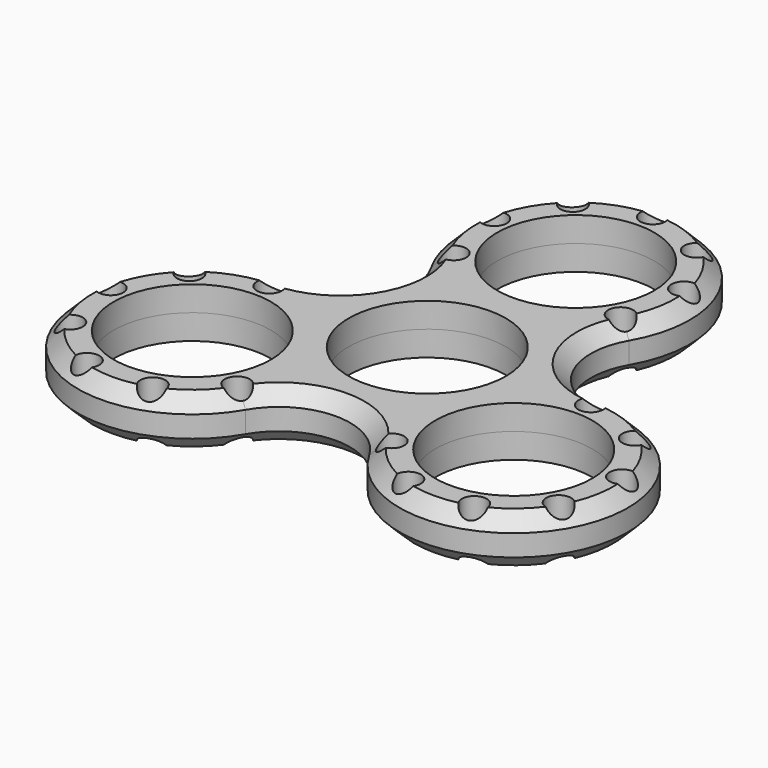
from build123d import *

# Parameters (mm, degrees)
F0_R         = 1.75
F0_R_2       = 11
F1_DEPTH     = 3.5
F2_T2_ANGLE  = 240
F2_T4_ANGLE  = 120
F2_T6_ANGLE  = 240
F2_T8_ANGLE  = 120
F2_T10_ANGLE = 240
F2_T12_ANGLE = 120
F2_T14_ANGLE = 120
F2_T16_ANGLE = 240
F2_T18_ANGLE = 120
F2_T20_ANGLE = 240
F2_T22_ANGLE = 120
F2_T24_ANGLE = 240


# Not quite as in the source:
# - a fillet or chamfer that OpenCascade refuses, or shapes differently, is made with other operations: its cross-section is extruded or revolved along the edge and cut away or added


with BuildPart() as f1:
    # F0 (on Top) → F1 (new body, symmetric)
    with BuildSketch(Plane.XY):
        with BuildLine():
            ThreePointArc((22.5166604984, 3), (13.8564064606, 8), (13.8564064606, 18))
            ThreePointArc((13.8564064606, 18), (0, 42), (-13.8564064606, 18))
            ThreePointArc((-13.8564064606, 18), (-13.8564064606, 8), (-22.5166604984, 3))
            ThreePointArc((-22.5166604984, 3), (-36.3730669589, -21), (-8.6602540378, -21))
            ThreePointArc((-8.6602540378, -21), (0, -16), (8.6602540378, -21))
            ThreePointArc((8.6602540378, -21), (36.3730669589, -21), (22.5166604984, 3))
        make_face()
        with Locations((-27.1339324333, -25.6858503806)):
            Circle(F0_R, mode=Mode.SUBTRACT)
        with Locations((-34.2080034495, -19.75)):
            Circle(F0_R, mode=Mode.SUBTRACT)
        with Locations((-22.5166604984, -13)):
            Circle(F0_R_2, mode=Mode.SUBTRACT)
        with Locations((-17.8993885635, -25.6858503806)):
            Circle(F0_R, mode=Mode.SUBTRACT)
        with Locations((-10.8253175473, -19.75)):
            Circle(F0_R, mode=Mode.SUBTRACT)
        with Locations((-35.8115651641, -10.6557496015)):
            Circle(F0_R, mode=Mode.SUBTRACT)
        with Locations((-31.1942932292, -2.6584000179)):
            Circle(F0_R, mode=Mode.SUBTRACT)
        with Locations((-22.5166604984, 0.5)):
            Circle(F0_R, mode=Mode.SUBTRACT)
        with Locations((17.8993885635, -25.6858503806)):
            Circle(F0_R, mode=Mode.SUBTRACT)
        with Locations((10.8253175473, -19.75)):
            Circle(F0_R, mode=Mode.SUBTRACT)
        with Locations((27.1339324333, -25.6858503806)):
            Circle(F0_R, mode=Mode.SUBTRACT)
        with Locations((22.5166604984, -13)):
            Circle(F0_R_2, mode=Mode.SUBTRACT)
        with Locations((34.2080034495, -19.75)):
            Circle(F0_R, mode=Mode.SUBTRACT)
        Circle(F0_R_2, mode=Mode.SUBTRACT)
        with Locations((35.8115651641, -10.6557496015)):
            Circle(F0_R, mode=Mode.SUBTRACT)
        with Locations((31.1942932292, -2.6584000179)):
            Circle(F0_R, mode=Mode.SUBTRACT)
        with Locations((22.5166604984, 0.5)):
            Circle(F0_R, mode=Mode.SUBTRACT)
        with BuildLine():
            ThreePointArc((-10.1480272234, 18.4249687492), (-13.4411094984, 19.221416266), (-10.1757984945, 20.125))
            ThreePointArc((-10.1757984945, 20.125), (-10.0009727551, 19.7029333289), (-9.9413429511, 19.25))
            ThreePointArc((-9.9413429511, 19.25), (-9.9938002383, 18.8247368599), (-10.1480272234, 18.4249687492))
        make_face(mode=Mode.SUBTRACT)
        with Locations((-13.2949046657, 28.3442503985)):
            Circle(F0_R, mode=Mode.SUBTRACT)
        with Locations((-8.6776327308, 36.3415999821)):
            Circle(F0_R, mode=Mode.SUBTRACT)
        with BuildLine():
            ThreePointArc((10.1480272234, 18.4249687492), (11.266079811, 20.9475427128), (13.4413429511, 19.25))
            ThreePointArc((13.4413429511, 19.25), (12.1166060911, 17.5524572872), (10.1480272234, 18.4249687492))
        make_face(mode=Mode.SUBTRACT)
        with BuildLine():
            ThreePointArc((-9.5262794416, 20.5), (-2.8470094961, 36.6251840892), (11, 26))
            ThreePointArc((11, 26), (2.8470094961, 15.3748159108), (-9.5262794416, 20.5))
        make_face(mode=Mode.SUBTRACT)
        with Locations((13.2949046657, 28.3442503985)):
            Circle(F0_R, mode=Mode.SUBTRACT)
        with Locations((8.6776327308, 36.3415999821)):
            Circle(F0_R, mode=Mode.SUBTRACT)
        with Locations((0, 39.5)):
            Circle(F0_R, mode=Mode.SUBTRACT)
    extrude(amount=F1_DEPTH, both=True)

    # F2: chamfer of 2 on 12 edges, made by hand

    # F2_s1 → F2_t2 (revolve, cut)
    with BuildSketch(Plane.YZ.offset(-22.5166604984)):
        Polygon((3, 1.5), (1, 3.5), (3, 3.5), align=None)
    revolve(axis=Axis((-22.5166604984, -13, 3.5), (0, 0, 1)), revolution_arc=F2_T2_ANGLE, mode=Mode.SUBTRACT)

    # F2_s3 → F2_t4 (revolve, cut)
    with BuildSketch(Plane(origin=(-11.2583302492, -19.5, 0), x_dir=(0, 0, 1), z_dir=(-0.5, -0.8660254038, 0))):
        Polygon((1.5, -3), (3.5, -1), (3.5, -3), align=None)
    revolve(axis=Axis((0, -26, 3.5), (0, 0, -1)), revolution_arc=F2_T4_ANGLE, mode=Mode.SUBTRACT)

    # F2_s5 → F2_t6 (revolve, cut)
    with BuildSketch(Plane(origin=(11.2583302492, -19.5, 0), x_dir=(0, 0, 1), z_dir=(-0.5, 0.8660254038, 0))):
        Polygon((1.5, -3), (3.5, -1), (3.5, -3), align=None)
    revolve(axis=Axis((22.5166604984, -13, 3.5), (0, 0, 1)), revolution_arc=F2_T6_ANGLE, mode=Mode.SUBTRACT)

    # F2_s7 → F2_t8 (revolve, cut)
    with BuildSketch(Plane.YZ.offset(22.5166604984)):
        Polygon((3, 1.5), (1, 3.5), (3, 3.5), align=None)
    revolve(axis=Axis((22.5166604984, 13, 3.5), (0, 0, -1)), revolution_arc=F2_T8_ANGLE, mode=Mode.SUBTRACT)

    # F2_s9 → F2_t10 (revolve, cut)
    with BuildSketch(Plane(origin=(11.2583302492, 19.5, 0), x_dir=(0, 0, 1), z_dir=(-0.5, -0.8660254038, 0))):
        Polygon((3.5, -1), (1.5, -3), (3.5, -3), align=None)
    revolve(axis=Axis((0, 26, 3.5), (0, 0, 1)), revolution_arc=F2_T10_ANGLE, mode=Mode.SUBTRACT)

    # F2_s11 → F2_t12 (revolve, cut)
    with BuildSketch(Plane(origin=(-11.2583302492, 19.5, 0), x_dir=(0, 0, 1), z_dir=(-0.5, 0.8660254038, 0))):
        Polygon((1.5, -3), (3.5, -1), (3.5, -3), align=None)
    revolve(axis=Axis((-22.5166604984, 13, 3.5), (0, 0, -1)), revolution_arc=F2_T12_ANGLE, mode=Mode.SUBTRACT)

    # F2_s13 → F2_t14 (revolve, cut)
    with BuildSketch(Plane(origin=(-11.2583302492, -19.5, 0), x_dir=(0, 0, 1), z_dir=(-0.5, -0.8660254038, 0))):
        Polygon((-1.5, -3), (-3.5, -1), (-3.5, -3), align=None)
    revolve(axis=Axis((0, -26, -3.5), (0, 0, -1)), revolution_arc=F2_T14_ANGLE, mode=Mode.SUBTRACT)

    # F2_s15 → F2_t16 (revolve, cut)
    with BuildSketch(Plane.YZ.offset(-22.5166604984)):
        Polygon((3, -1.5), (1, -3.5), (3, -3.5), align=None)
    revolve(axis=Axis((-22.5166604984, -13, -3.5), (0, 0, 1)), revolution_arc=F2_T16_ANGLE, mode=Mode.SUBTRACT)

    # F2_s17 → F2_t18 (revolve, cut)
    with BuildSketch(Plane(origin=(-11.2583302492, 19.5, 0), x_dir=(0, 0, 1), z_dir=(-0.5, 0.8660254038, 0))):
        Polygon((-1.5, -3), (-3.5, -1), (-3.5, -3), align=None)
    revolve(axis=Axis((-22.5166604984, 13, -3.5), (0, 0, -1)), revolution_arc=F2_T18_ANGLE, mode=Mode.SUBTRACT)

    # F2_s19 → F2_t20 (revolve, cut)
    with BuildSketch(Plane(origin=(11.2583302492, 19.5, 0), x_dir=(0, 0, 1), z_dir=(-0.5, -0.8660254038, 0))):
        Polygon((-1.5, -3), (-3.5, -1), (-3.5, -3), align=None)
    revolve(axis=Axis((0, 26, -3.5), (0, 0, 1)), revolution_arc=F2_T20_ANGLE, mode=Mode.SUBTRACT)

    # F2_s21 → F2_t22 (revolve, cut)
    with BuildSketch(Plane.YZ.offset(22.5166604984)):
        Polygon((3, -1.5), (1, -3.5), (3, -3.5), align=None)
    revolve(axis=Axis((22.5166604984, 13, -3.5), (0, 0, -1)), revolution_arc=F2_T22_ANGLE, mode=Mode.SUBTRACT)

    # F2_s23 → F2_t24 (revolve, cut)
    with BuildSketch(Plane(origin=(11.2583302492, -19.5, 0), x_dir=(0, 0, 1), z_dir=(-0.5, 0.8660254038, 0))):
        Polygon((-1.5, -3), (-3.5, -1), (-3.5, -3), align=None)
    revolve(axis=Axis((22.5166604984, -13, -3.5), (0, 0, 1)), revolution_arc=F2_T24_ANGLE, mode=Mode.SUBTRACT)


solid = f1.part
